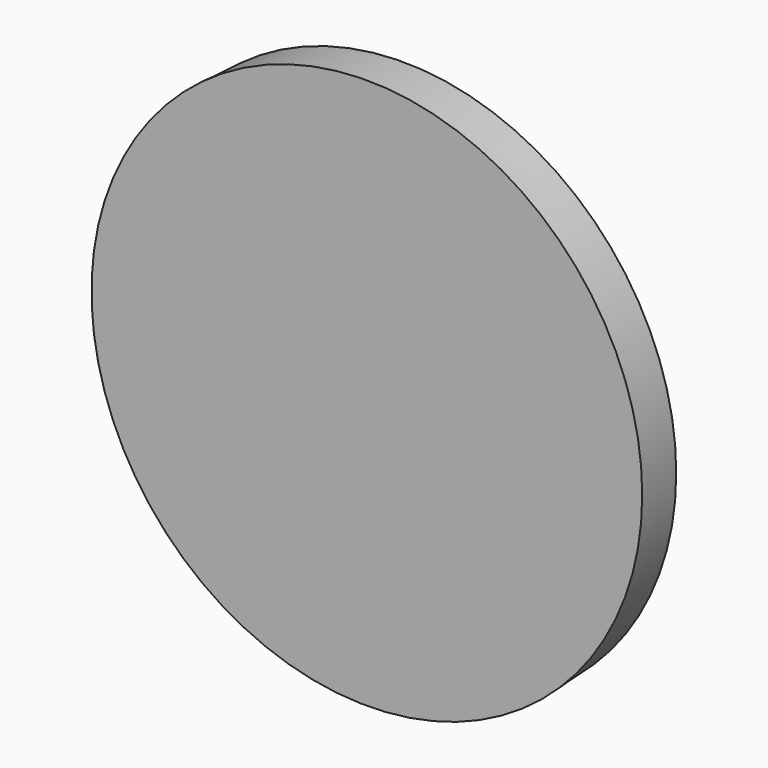
from build123d import *

# Parameters (mm, degrees)
F0_R     = 15
F1_DEPTH = 51.7
F1_TAPER = -3
F2_T     = -2.5


with BuildPart() as f1:
    # F0 (on Front) → F1 (new body)
    with BuildSketch(Plane.XZ):
        Circle(F0_R)
    extrude(amount=F1_DEPTH, taper=F1_TAPER)

    # F2
    f2_openings = [f1.faces().sort_by_distance(p)[0] for p in [
        (0, -51.7, 0),
        (-16.354741, -25.85, 0),
    ]]
    offset(amount=F2_T, openings=f2_openings)


solid = f1.part
